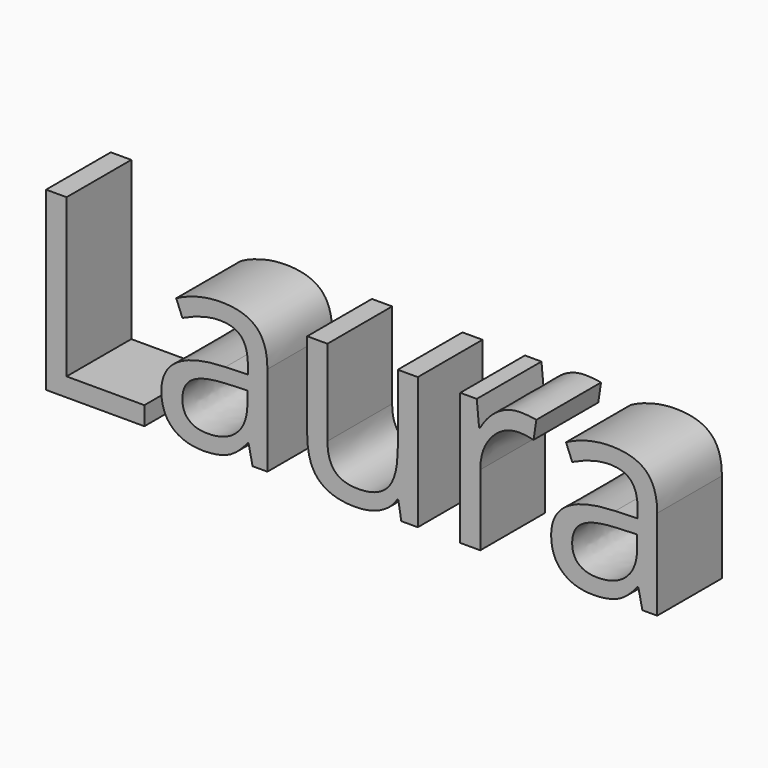
from build123d import *

# Parameters (mm, degrees)
F0_TEXT_SIZE = 76.3544295397
F1_DEPTH     = 25


# Not quite as in the source:
# - Text() gives the source's letters only with a copy of the font that has no kerning and outlines rounded to 1/6400 em; it was checked with that copy


with BuildPart() as f1:
    # F0 (on Front) → F1 (new body)
    with BuildSketch(Plane.XZ):
        with Locations((-100.766133517, -27.3573212326)):
            Text('Laura', F0_TEXT_SIZE, font='Open Sans', text_align=(TextAlign.LEFT, TextAlign.BOTTOM))
    extrude(amount=F1_DEPTH)


solid = f1.part
